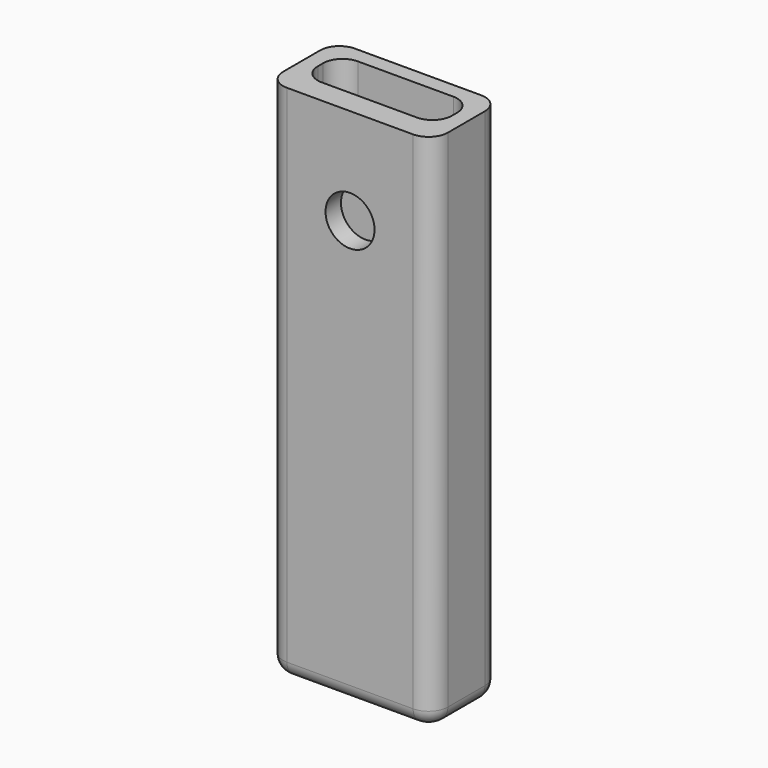
from build123d import *

# Parameters (mm, degrees)
F0_W     = 27.1145
F0_H     = 13.97
F0_W_2   = 22.0345
F0_H_2   = 7.46125
F1_DEPTH = 42.8625
F2_R     = 3.175
F3_R     = 4.03225
F4_DEPTH = 3.175
F6_DEPTH = 0.3175
F7_R     = 2.54


with BuildPart() as f1:
    # F0 (on Top) → F1 (new body, symmetric)
    with BuildSketch(Plane.XY):
        Rectangle(F0_W, F0_H)
        with Locations((0, 0.714375)):
            Rectangle(F0_W_2, F0_H_2, mode=Mode.SUBTRACT)
    extrude(amount=F1_DEPTH, both=True)

    # F2
    f2_edges = [f1.edges().sort_by_distance(p)[0] for p in [
        (13.55725, -6.985, 0),
        (-13.55725, -6.985, 0),
        (-13.55725, 6.985, 0),
        (13.55725, 6.985, 0),
        (-11.01725, 4.445, 0),
        (11.01725, 4.445, 0),
        (11.01725, -3.01625, 0),
        (-11.01725, -3.01625, 0),
    ]]
    fillet(f2_edges, radius=F2_R)

    # F3 (on face) → F4 (cut)
    with BuildSketch(Plane.XZ.offset(6.985)):
        with Locations((0, 26.9875)):
            Circle(F3_R)
    extrude(amount=-F4_DEPTH, mode=Mode.SUBTRACT)

    # F5 (on face) → F6 (join)
    with BuildSketch(Plane(origin=(0, 0, -42.8625), x_dir=(1, 0, 0), z_dir=(0, 0, -1))):
        with BuildLine():
            ThreePointArc((11.01725, -0.15875), (10.0873140303, 2.0863140303), (7.84225, 3.01625))
            Line((7.84225, 3.01625), (-7.84225, 3.01625))
            ThreePointArc((-7.84225, 3.01625), (-10.0873140303, 2.0863140303), (-11.01725, -0.15875))
            Line((-11.01725, -0.15875), (-11.01725, -1.27))
            ThreePointArc((-11.01725, -1.27), (-10.0873140303, -3.5150640303), (-7.84225, -4.445))
            Line((-7.84225, -4.445), (7.84225, -4.445))
            ThreePointArc((7.84225, -4.445), (10.0873140303, -3.5150640303), (11.01725, -1.27))
            Line((11.01725, -1.27), (11.01725, -0.15875))
        make_face()
    extrude(amount=-F6_DEPTH)

    # F7
    f7_edges = [f1.edges().sort_by_distance(p)[0] for p in [
        (0, -6.985, -42.8625),
        (12.627314, -6.055064, -42.8625),
        (13.55725, 0, -42.8625),
        (12.627314, 6.055064, -42.8625),
        (0, 6.985, -42.8625),
        (-12.627314, 6.055064, -42.8625),
        (-13.55725, 0, -42.8625),
        (-12.627314, -6.055064, -42.8625),
    ]]
    fillet(f7_edges, radius=F7_R)


solid = f1.part
